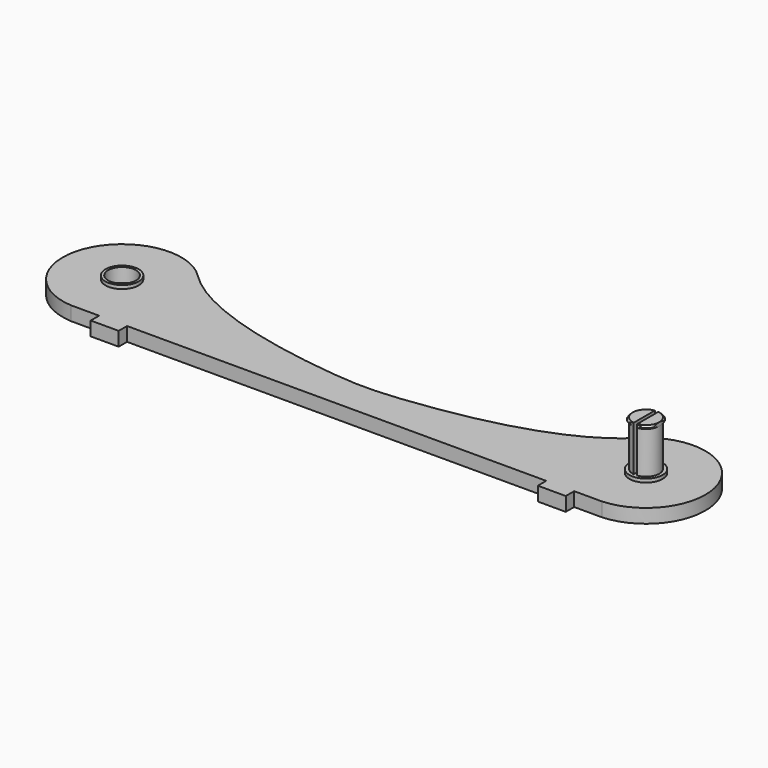
from build123d import *

# Parameters (mm, degrees)
F2_DEPTH  = 4
F3_R      = 3.8
F4_DEPTH  = 13
F5_R      = 3.8
F6_DEPTH  = 0.5
F6_TAPER  = -45
F7_R      = 4.3
F8_DEPTH  = 0.5
F8_TAPER  = 45
F9_W      = 1
F9_H      = 11
F10_DEPTH = 13
F11_R     = 4
F12_DEPTH = 3
F13_R     = 4
F14_DEPTH = 0.5
F14_TAPER = -45
F15_DEPTH = 0.5
F16_R     = 4.75
F16_R_2   = 4
F16_R_3   = 3.8
F17_DEPTH = 1
F18_W     = 11.6
F18_H     = 11.6
F19_DEPTH = 5


with BuildPart() as f2:
    # F1 (on Top) → F2 (new body)
    with BuildSketch(Plane.XY):
        with BuildLine():
            add(Edge.make_bspline(
                [(-62.9584054212, 12), (-50.9998563223, 0), (-9.8574829598, -7.14219171), (9.8574829598, -7.14219171), (50.9998563223, 0), (62.9584054212, 12)],
                knots=[0, 0, 0, 0, 0.3750382163, 0.6249617837, 1, 1, 1, 1], degree=3))
            ThreePointArc((-62.9584054212, 12), (-90.5016960105, 6.9783537313), (-76, -16.9705627485))
            Line((-76, -16.9705627485), (-68, -16.9705627485))
            Line((-68, -16.9705627485), (-68, -19.9705627485))
            Line((-68, -19.9705627485), (-60, -19.9705627485))
            Line((-60, -19.9705627485), (-60, -16.9705627485))
            Line((-60, -16.9705627485), (60, -16.9705627485))
            Line((60, -16.9705627485), (60, -19.9705627485))
            Line((60, -19.9705627485), (68, -19.9705627485))
            Line((68, -19.9705627485), (68, -16.9705627485))
            Line((68, -16.9705627485), (76, -16.9705627485))
            ThreePointArc((76, -16.9705627485), (90.5016960105, 6.9783537313), (62.9584054212, 12))
        make_face()
    extrude(amount=F2_DEPTH)

    # F3 (on face) → F4 (join)
    with BuildSketch(Plane.XY.offset(4)):
        with Locations((75, 0)):
            Circle(F3_R)
    extrude(amount=F4_DEPTH)

    # F5 (on face) → F6 (join)
    with BuildSketch(Plane.XY.offset(17)):
        with Locations((75, 0)):
            Circle(F5_R)
    extrude(amount=F6_DEPTH, taper=F6_TAPER)

    # F7 (on face) → F8 (join)
    with BuildSketch(Plane.XY.offset(17.5)):
        with Locations((75, 0)):
            Circle(F7_R)
    extrude(amount=F8_DEPTH, taper=F8_TAPER)

    # F9 (on face) → F10 (cut)
    with BuildSketch(Plane.XY.offset(18)):
        with Locations((75, 0)):
            Rectangle(F9_W, F9_H)
    extrude(amount=-F10_DEPTH, mode=Mode.SUBTRACT)

    # F11 (on face) → F12 (cut)
    with BuildSketch(Plane.XY.offset(4)):
        with Locations((-75, 0)):
            Circle(F11_R)
    extrude(amount=-F12_DEPTH, mode=Mode.SUBTRACT)

    # F13 (on face) → F14 (cut)
    with BuildSketch(Plane.XY.offset(1)):
        with Locations((-75, 0)):
            Circle(F13_R)
    extrude(amount=-F14_DEPTH, taper=F14_TAPER, mode=Mode.SUBTRACT)

    # F15 (cut): a face of the model
    f15_faces = [f2.faces().sort_by_distance(p)[0] for p in [
        (-75, 0, 0.5),
    ]]
    extrude(f15_faces, amount=-F15_DEPTH, mode=Mode.SUBTRACT)

    # F16 (on face) → F17 (join)
    with BuildSketch(Plane.XY.offset(4)):
        with Locations((-75, 0)):
            Circle(F16_R)
        with Locations((-75, 0)):
            Circle(F16_R_2, mode=Mode.SUBTRACT)
        with Locations((75, 0)):
            Circle(F16_R)
        with Locations((75, 0)):
            Circle(F16_R_3, mode=Mode.SUBTRACT)
    extrude(amount=F17_DEPTH)

    # F18 (on face) → F19 (cut)
    with BuildSketch(Plane.XY.offset(18)):
        with Locations((75, 0)):
            Rectangle(F18_W, F18_H)
        Polygon((71.2, 0), (71.2, 3.8), (78.8, 3.8), (78.8, -3.8), (71.2, -3.8), align=None, mode=Mode.SUBTRACT)
    extrude(amount=-F19_DEPTH, mode=Mode.SUBTRACT)


solid = f2.part
